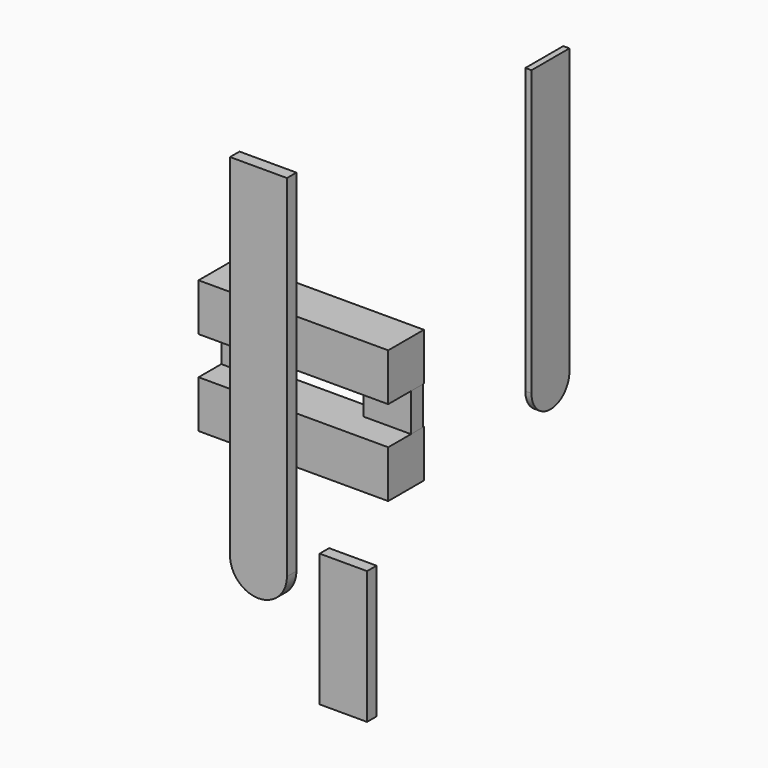
from build123d import *

# Parameters (mm, degrees)
F0_W          = 12.7
F0_H          = 12.7
F0_W_2        = 25.4
F1_DEPTH      = 7.62
F1_DEPTH_BACK = 4.318
F0_H_2        = 10.16
F2_DEPTH      = 4.064
F3_W          = 15.24
F3_H          = 12.7
F3_H_2        = 56.7852711724
F4_DEPTH      = 3.175
F6_DEPTH      = 1.651
F7_W          = 12.7
F7_H          = 35.56
F8_DEPTH      = 3.175


# Not quite as in the source:
# - a length typed as a fraction of an inch, garbled in the dataset ("3 / 203.2 mm" for 3/8 in), is restored
# - a feature names something its author has since deleted; it is built from what else it names


with BuildPart() as f1:
    # F0 (on Front) → F1 (new body, two sides)
    with BuildSketch(Plane.XZ) as f1_sk:
        with Locations((-11.6530044077, 29.21)):
            Rectangle(F0_W, F0_H)
        with Locations((-30.7030044077, 29.21)):
            Rectangle(F0_W_2, F0_H)
        with Locations((-49.7530044077, 29.21)):
            Rectangle(F0_W, F0_H)
    extrude(amount=F1_DEPTH)
    extrude(f1_sk.sketch, amount=-F1_DEPTH_BACK)


with BuildPart() as f1b:
    # F0 (on Front) → F1, piece 2 (new body, two sides)
    with BuildSketch(Plane.XZ) as f1_2_sk:
        with Locations((-49.7530044077, 6.35)):
            Rectangle(F0_W, F0_H)
        with Locations((-30.7030044077, 6.35)):
            Rectangle(F0_W_2, F0_H)
        with Locations((-11.6530044077, 6.35)):
            Rectangle(F0_W, F0_H)
    extrude(amount=F1_DEPTH)
    extrude(f1_2_sk.sketch, amount=-F1_DEPTH_BACK)


with BuildPart() as f2:
    # F0 (on Front) → F2 (new body)
    with BuildSketch(Plane.XZ):
        with Locations((-11.6530044077, 17.78)):
            Rectangle(F0_W, F0_H_2)
    extrude(amount=-F2_DEPTH)


with BuildPart() as f2b:
    # F0 (on Front) → F2, piece 2 (new body)
    with BuildSketch(Plane.XZ):
        with Locations((-49.7530044077, 17.78)):
            Rectangle(F0_W, F0_H_2)
    extrude(amount=-F2_DEPTH)


with BuildPart() as f4:
    # F3 (on face) → F4 (new body)
    with BuildSketch(Plane.XZ.offset(7.62)):
        with BuildLine():
            ThreePointArc((-45.1375190453, -24.4947288276), (-37.5175190453, -32.1147288276), (-29.8975190453, -24.4947288276))
            Line((-29.8975190453, -24.4947288276), (-29.8975190453, 0))
            Line((-29.8975190453, 0), (-45.1375190453, 0))
            Line((-45.1375190453, 0), (-45.1375190453, -24.4947288276))
        make_face()
        with Locations((-37.5175190453, 6.35)):
            Rectangle(F3_W, F3_H)
        with Locations((-37.5175190453, 41.0926355862)):
            Rectangle(F3_W, F3_H_2)
    extrude(amount=F4_DEPTH)


with BuildPart() as f6:
    # F5 (on Right) → F6 (new body)
    with BuildSketch(Plane.YZ):
        with BuildLine():
            Line((44.3628823752, 87.9049419045), (31.6628823752, 87.9049419045))
            Line((31.6628823752, 87.9049419045), (31.6628823752, 11.7049419045))
            ThreePointArc((31.6628823752, 11.7049419045), (38.0128823752, 5.3549419045), (44.3628823752, 11.7049419045))
            Line((44.3628823752, 11.7049419045), (44.3628823752, 87.9049419045))
        make_face()
    extrude(amount=F6_DEPTH)


with BuildPart() as f8:
    # F7 (on Front) → F8 (new body)
    with BuildSketch(Plane.XZ):
        with Locations((-20.8775842459, -39.0941523947)):
            Rectangle(F7_W, F7_H)
    extrude(amount=F8_DEPTH)


solid = Compound([f1.part, f1b.part, f2.part, f2b.part, f4.part, f6.part, f8.part])
